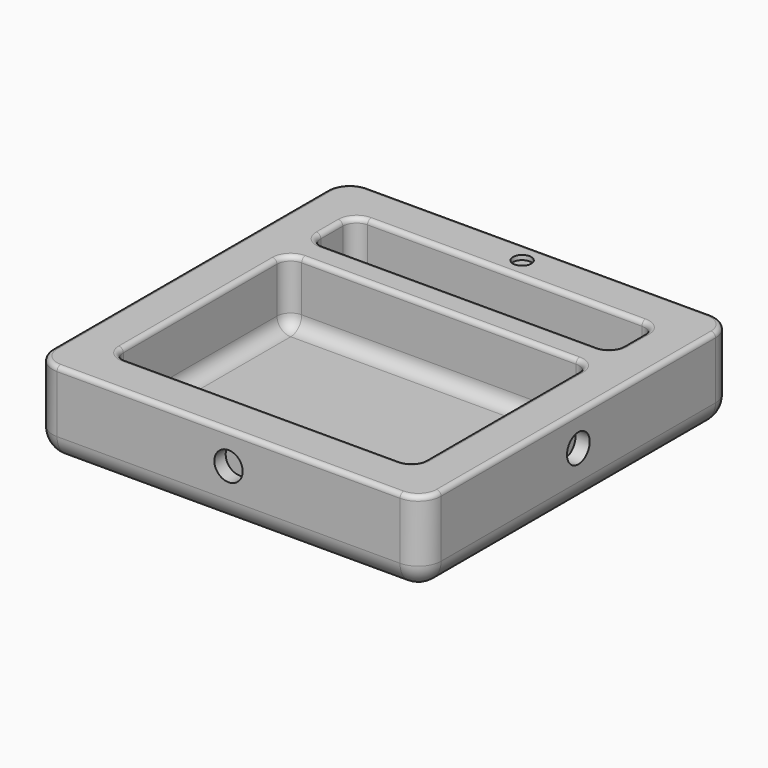
from build123d import *

# Parameters (mm, degrees)
F0_W      = 85
F0_H      = 85
F0_R      = 2
F3_DEPTH  = 18.5
F4_DEPTH  = 14
F5_R      = 5
F6_R      = 3
F7_R      = 1
F8_R      = 3.1
F9_DEPTH  = 3.1
F10_R     = 3.1
F11_DEPTH = 3.1
F12_R     = 3.1
F13_DEPTH = 3.1
F14_R     = 3.1
F15_DEPTH = 3.1
F16_DEPTH = 1
F17_ANGLE = 180


# Not quite as in the source:
# - a feature names something its author has since deleted; it is built from what else it names


with BuildPart() as f3:
    # F0 (on Top) → F3 (new body)
    with BuildSketch(Plane.XY):
        Rectangle(F0_W, F0_H)
        with BuildLine():
            ThreePointArc((-33, 12), (-32.1213203436, 14.1213203436), (-30, 15))
            Line((-30, 15), (30, 15))
            ThreePointArc((30, 15), (32.1213203436, 14.1213203436), (33, 12))
            Line((33, 12), (33, -30))
            ThreePointArc((33, -30), (32.1213203436, -32.1213203436), (30, -33))
            Line((30, -33), (-30, -33))
            ThreePointArc((-30, -33), (-32.1213203436, -32.1213203436), (-33, -30))
            Line((-33, -30), (-33, 12))
        make_face(mode=Mode.SUBTRACT)
        with BuildLine():
            ThreePointArc((-33, 30), (-32.1213203436, 32.1213203436), (-30, 33))
            Line((-30, 33), (30, 33))
            ThreePointArc((30, 33), (32.1213203436, 32.1213203436), (33, 30))
            Line((33, 30), (33, 24))
            ThreePointArc((33, 24), (32.1213203436, 21.8786796564), (30, 21))
            Line((30, 21), (-30, 21))
            ThreePointArc((-30, 21), (-32.1213203436, 21.8786796564), (-33, 24))
            Line((-33, 24), (-33, 30))
        make_face(mode=Mode.SUBTRACT)
        with Locations((0, 37.75)):
            Circle(F0_R, mode=Mode.SUBTRACT)
        with BuildLine():
            Line((30, 15), (-30, 15))
            ThreePointArc((-30, 15), (-32.1213203436, 14.1213203436), (-33, 12))
            Line((-33, 12), (-33, -30))
            ThreePointArc((-33, -30), (-32.1213203436, -32.1213203436), (-30, -33))
            Line((-30, -33), (30, -33))
            ThreePointArc((30, -33), (32.1213203436, -32.1213203436), (33, -30))
            Line((33, -30), (33, 12))
            ThreePointArc((33, 12), (32.1213203436, 14.1213203436), (30, 15))
        make_face()
        with BuildLine():
            Line((30, 33), (-30, 33))
            ThreePointArc((-30, 33), (-32.1213203436, 32.1213203436), (-33, 30))
            Line((-33, 30), (-33, 24))
            ThreePointArc((-33, 24), (-32.1213203436, 21.8786796564), (-30, 21))
            Line((-30, 21), (30, 21))
            ThreePointArc((30, 21), (32.1213203436, 21.8786796564), (33, 24))
            Line((33, 24), (33, 30))
            ThreePointArc((33, 30), (32.1213203436, 32.1213203436), (30, 33))
        make_face()
        with Locations((0, 37.75)):
            Circle(F0_R)
    extrude(amount=F3_DEPTH)

    # F0 (on Top) → F4 (cut)
    with BuildSketch(Plane.XY):
        with BuildLine():
            Line((30, 33), (-30, 33))
            ThreePointArc((-30, 33), (-32.1213203436, 32.1213203436), (-33, 30))
            Line((-33, 30), (-33, 24))
            ThreePointArc((-33, 24), (-32.1213203436, 21.8786796564), (-30, 21))
            Line((-30, 21), (30, 21))
            ThreePointArc((30, 21), (32.1213203436, 21.8786796564), (33, 24))
            Line((33, 24), (33, 30))
            ThreePointArc((33, 30), (32.1213203436, 32.1213203436), (30, 33))
        make_face()
        with BuildLine():
            Line((30, 15), (-30, 15))
            ThreePointArc((-30, 15), (-32.1213203436, 14.1213203436), (-33, 12))
            Line((-33, 12), (-33, -30))
            ThreePointArc((-33, -30), (-32.1213203436, -32.1213203436), (-30, -33))
            Line((-30, -33), (30, -33))
            ThreePointArc((30, -33), (32.1213203436, -32.1213203436), (33, -30))
            Line((33, -30), (33, 12))
            ThreePointArc((33, 12), (32.1213203436, 14.1213203436), (30, 15))
        make_face()
    extrude(amount=F4_DEPTH, mode=Mode.SUBTRACT)

    # F5
    f5_edges = [f3.edges().sort_by_distance(p)[0] for p in [
        (0, 42.5, 18.5),
        (-42.5, 0, 18.5),
        (0, -42.5, 18.5),
        (42.5, 0, 18.5),
        (42.5, 42.5, 9.25),
        (-42.5, 42.5, 9.25),
        (-42.5, -42.5, 9.25),
        (42.5, -42.5, 9.25),
    ]]
    fillet(f5_edges, radius=F5_R)

    # F6
    f6_edges = [f3.edges().sort_by_distance(p)[0] for p in [
        (0, 33, 14),
        (-32.12132, 32.12132, 14),
        (-33, 27, 14),
        (-32.12132, 21.87868, 14),
        (0, 21, 14),
        (32.12132, 21.87868, 14),
        (33, 27, 14),
        (32.12132, 32.12132, 14),
        (0, 15, 14),
        (-32.12132, 14.12132, 14),
        (-33, -9, 14),
        (-32.12132, -32.12132, 14),
        (0, -33, 14),
        (32.12132, -32.12132, 14),
        (33, -9, 14),
        (32.12132, 14.12132, 14),
    ]]
    fillet(f6_edges, radius=F6_R)

    # F7
    f7_edges = [f3.edges().sort_by_distance(p)[0] for p in [
        (0, 42.5, 0),
        (41.035534, 41.035534, 0),
        (-41.035534, 41.035534, 0),
        (42.5, 0, 0),
        (-42.5, 0, 0),
        (41.035534, -41.035534, 0),
        (-41.035534, -41.035534, 0),
        (0, -42.5, 0),
        (0, 15, 0),
        (-32.12132, 14.12132, 0),
        (-33, -9, 0),
        (-32.12132, -32.12132, 0),
        (0, -33, 0),
        (32.12132, -32.12132, 0),
        (33, -9, 0),
        (32.12132, 14.12132, 0),
        (0, 33, 0),
        (-32.12132, 32.12132, 0),
        (-33, 27, 0),
        (-32.12132, 21.87868, 0),
        (0, 21, 0),
        (32.12132, 21.87868, 0),
        (33, 27, 0),
        (32.12132, 32.12132, 0),
    ]]
    fillet(f7_edges, radius=F7_R)

    # F8 (on face) → F9 (cut)
    with BuildSketch(Plane.XZ.offset(42.5)):
        with Locations((0, 7)):
            Circle(F8_R)
    extrude(amount=-F9_DEPTH, mode=Mode.SUBTRACT)

    # F10 (on face) → F11 (cut)
    with BuildSketch(Plane(origin=(0, 42.5, 0), x_dir=(-1, 0, 0), z_dir=(0, 1, 0))):
        with Locations((0, 7)):
            Circle(F10_R)
    extrude(amount=-F11_DEPTH, mode=Mode.SUBTRACT)

    # F12 (on face) → F13 (cut)
    with BuildSketch(Plane(origin=(-42.5, 0, 0), x_dir=(0, -1, 0), z_dir=(-1, 0, 0))):
        with Locations((0, 7)):
            Circle(F12_R)
    extrude(amount=-F13_DEPTH, mode=Mode.SUBTRACT)

    # F14 (on face) → F15 (cut)
    with BuildSketch(Plane.YZ.offset(42.5)):
        with Locations((0, 7)):
            Circle(F14_R)
    extrude(amount=-F15_DEPTH, mode=Mode.SUBTRACT)

    # F0 (on Top) → F16 (cut)
    with BuildSketch(Plane.XY):
        with Locations((0, 37.75)):
            Circle(F0_R)
    extrude(amount=F16_DEPTH, mode=Mode.SUBTRACT)


with BuildPart() as f3_1:
    # F17: moved
    add(f3.part.rotate(Axis((0, 0, 0), (0, 1, 0)), F17_ANGLE))


solid = f3_1.part
